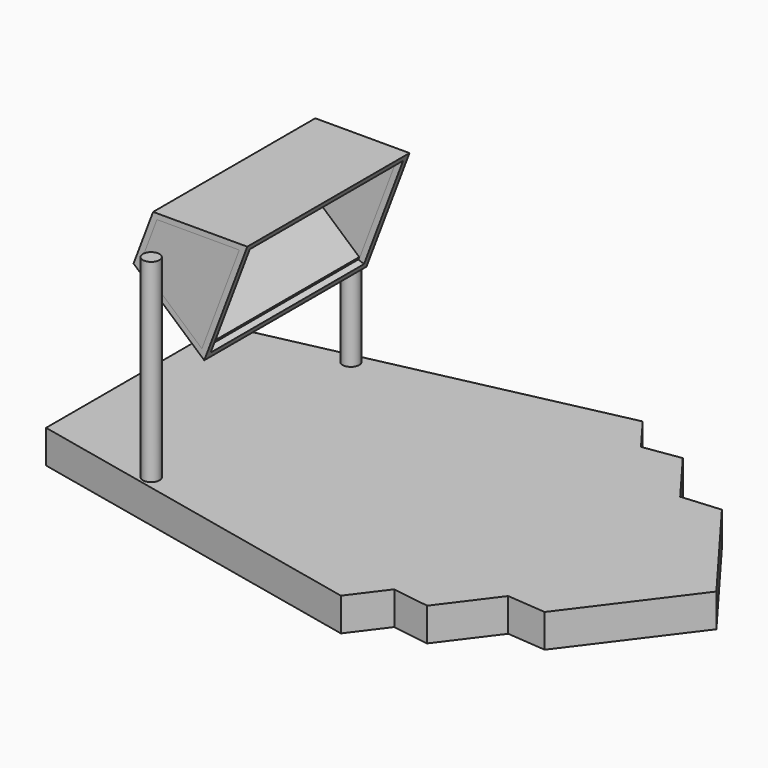
from build123d import *

# Parameters (mm, degrees)
F1_DEPTH  = 6
F4_R      = 1.5
F5_DEPTH  = 35
F12_DEPTH = 1
F14_DEPTH = 36.6
F15_W     = 34.6
F15_H     = 20
F16_DEPTH = 1.1
F17_DEPTH = 39.7
F18_DEPTH = 40.4


# Not quite as in the source:
# - a feature of the source that left no trace in its solid (it failed there, or was rolled back) is left out
# - the program builds the solid bodies; features that only make, move or delete a surface that nothing else refers to are left out


with BuildPart() as f1:
    # F0 (on Top) → F1 (new body)
    with BuildSketch(Plane.XY):
        Polygon((37.9445583731, -19.4072555025), (45, -20), (60, 0), (-45, 0), (-45, -12.4388851051), align=None)
        Polygon((30.8642615863, -28.8476512183), (37.9445583731, -19.4072555025), (-45, -12.4388851051), (-45, -17.4388851051), (24.1244330356, -27.8340892858), align=None)
        Polygon((24.1244330356, -27.8340892858), (-45, -17.4388851051), (-45, -20), (19.4574833105, -34.0566889193), align=None)
    extrude(amount=F1_DEPTH)

    # F2: F1 across plane


with BuildPart() as f1_1:
    add(f1.part)
    add(f1.part.mirror(Plane.XZ))

    # F4 (on face) → F5 (join)
    with BuildSketch(Plane.XY.offset(6)):
        with Locations((-24, -22.5326099851)):
            Circle(F4_R)
        with Locations((-24, 22.5326099851)):
            Circle(F4_R)
    extrude(amount=F5_DEPTH)

    # F17 (add): a face of the model
    f17_faces = [f1_1.faces().sort_by_distance(p)[0] for p in [
        (-24, -22.5326099851, 41),
    ]]
    extrude(f17_faces, amount=-F17_DEPTH)

    # F18 (add): a face of the model
    f18_faces = [f1_1.faces().sort_by_distance(p)[0] for p in [
        (-24, 22.5326099851, 41),
    ]]
    extrude(f18_faces, amount=-F18_DEPTH)


with BuildPart() as f12:
    # F11 (on offset) → F12 (new body)
    with BuildSketch(Plane.XZ.offset(-18.3)):
        Polygon((-10.0405558896, 45.4629359559), (-27.0405558896, 45.4629359559), (-30.5699676544, 36.1064808262), (-17.805261772, 24.8787346705), align=None)
        Polygon((-29.3902407032, 36.4005984732), (-26.3489918148, 44.4629359559), (-11.4865535006, 44.4629359559), (-18.230555187, 26.5846170234), align=None, mode=Mode.SUBTRACT)
        Polygon((-11.4865535006, 44.4629359559), (-26.3489918148, 44.4629359559), (-29.3902407032, 36.4005984732), (-18.230555187, 26.5846170234), align=None)
    extrude(amount=F12_DEPTH)


with BuildPart() as f13_1:
    # F13: instance of F12
    add(f12.part.mirror(Plane.XZ))


with BuildPart() as f14:
    # F11 (on offset) → F14 (new body, through all)
    with BuildSketch(Plane.XZ.offset(-18.3)):
        Polygon((-10.0405558896, 45.4629359559), (-27.0405558896, 45.4629359559), (-30.5699676544, 36.1064808262), (-17.805261772, 24.8787346705), align=None)
        Polygon((-29.3902407032, 36.4005984732), (-26.3489918148, 44.4629359559), (-11.4865535006, 44.4629359559), (-18.230555187, 26.5846170234), align=None, mode=Mode.SUBTRACT)
    extrude(amount=F14_DEPTH)

    # F15 (on face) → F16 (cut)
    with BuildSketch(Plane(origin=(-23.8029558046, 0, 8.9788740593), x_dir=(0, 1, 0), z_dir=(0.935645513, 0, -0.3529411765))):
        with Locations((0, 27.9934664258)):
            Rectangle(F15_W, F15_H)
    extrude(amount=-F16_DEPTH, mode=Mode.SUBTRACT)


solid = Compound([f1_1.part, f12.part, f13_1.part, f14.part])
